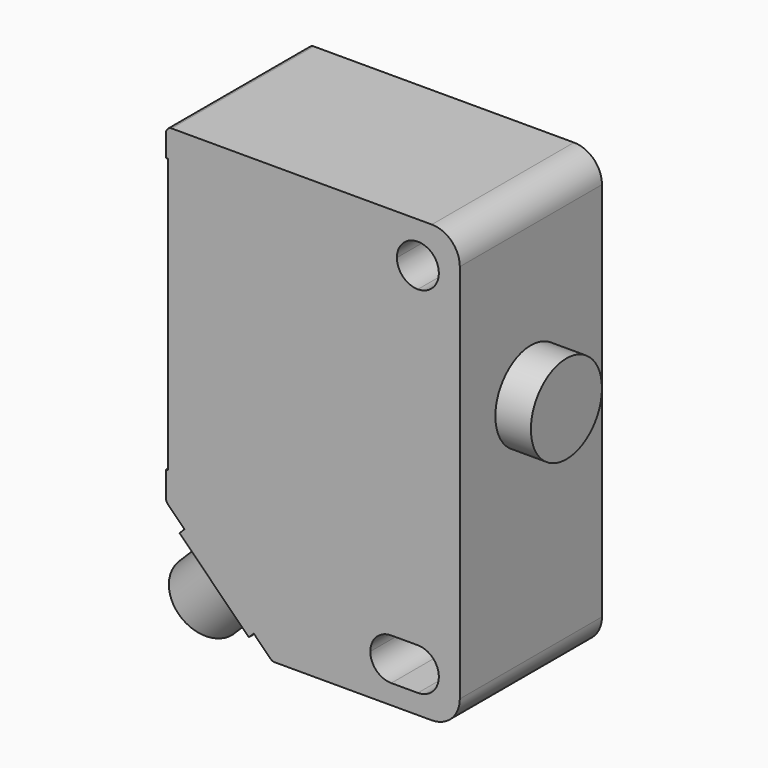
from build123d import *

# Parameters (mm, degrees)
F1_DEPTH = 12.7
F2_R     = 2.54
F3_DEPTH = 7.62
F4_R     = 3.175
F5_DEPTH = 2.54


# Not quite as in the source:
# - ends of sketch curves that miss each other by under 0.0002 mm in the source are joined


with BuildPart() as f1:
    # F0 (on Front) → F1 (new body)
    with BuildSketch(Plane.XZ):
        with BuildLine():
            Line((-46.1111856, 159.2312536), (-64.7111856, 159.2312536))
            ThreePointArc((-64.7111856, 159.2312536), (-64.9940283125, 159.1140963125), (-65.1111856, 158.8312536))
            Line((-65.1111856, 158.8312536), (-65.1111856, 157.2332636))
            Line((-65.1111856, 157.2332636), (-64.9611856, 157.2332636))
            Line((-64.9611856, 157.2332636), (-64.9611856, 137.6312536))
            Line((-64.9611856, 137.6312536), (-65.1111856, 137.6312536))
            Line((-65.1111856, 137.6312536), (-65.1111856, 135.7900576))
            ThreePointArc((-65.1111856, 135.7900576), (-65.080737413, 135.6369842271), (-64.9940283125, 135.5072148875))
            Line((-64.9940283125, 135.5072148875), (-63.7917726, 134.3049586))
            Line((-63.7917726, 134.3049586), (-64.1453256, 133.9514056))
            Line((-64.1453256, 133.9514056), (-63.6715641479, 133.4776440521))
            Line((-63.6715641479, 133.4776440521), (-59.6693400521, 129.4754191479))
            Line((-59.6693400521, 129.4754191479), (-59.1955786, 129.0016576))
            Line((-59.1955786, 129.0016576), (-58.8420246, 129.3552116))
            Line((-58.8420246, 129.3552116), (-57.6352246, 128.1484116))
            ThreePointArc((-57.6352246, 128.1484116), (-57.5054559729, 128.061701787), (-57.3523826, 128.0312536))
            Line((-57.3523826, 128.0312536), (-46.1111856, 128.0312536))
            ThreePointArc((-46.1111856, 128.0312536), (-44.6969720376, 128.6170400376), (-44.1111856, 130.0312536))
            Line((-44.1111856, 130.0312536), (-44.1111856, 134.1120546))
            Line((-44.1111856, 134.1120546), (-44.1111856, 153.1264526))
            Line((-44.1111856, 153.1264526), (-44.1111856, 156.3312536))
            Line((-44.1111856, 156.3312536), (-44.1111856, 157.2312536))
            ThreePointArc((-44.1111856, 157.2312536), (-44.6969720376, 158.6454671624), (-46.1111856, 159.2312536))
        make_face()
        with BuildLine():
            Line((-49.0111856, 132.4312536), (-47.1111856, 132.4312536))
            ThreePointArc((-47.1111856, 132.4312536), (-46.0505254282, 131.9919137718), (-45.6111856, 130.9312536))
            ThreePointArc((-45.6111856, 130.9312536), (-46.0505254282, 129.8705934282), (-47.1111856, 129.4312536))
            Line((-47.1111856, 129.4312536), (-49.0111856, 129.4312536))
            ThreePointArc((-49.0111856, 129.4312536), (-50.0718457718, 129.8705934282), (-50.5111856, 130.9312536))
            ThreePointArc((-50.5111856, 130.9312536), (-50.0718457718, 131.9919137718), (-49.0111856, 132.4312536))
        make_face(mode=Mode.SUBTRACT)
        with BuildLine():
            ThreePointArc((-47.1111856, 157.8312536), (-46.0505254282, 157.3919137718), (-45.6111856, 156.3312536))
            ThreePointArc((-45.6111856, 156.3312536), (-46.0505254282, 155.2705934282), (-47.1111856, 154.8312536))
            ThreePointArc((-47.1111856, 154.8312536), (-48.1718457718, 155.2705934282), (-48.6111856, 156.3312536))
            ThreePointArc((-48.6111856, 156.3312536), (-48.1718457718, 157.3919137718), (-47.1111856, 157.8312536))
        make_face(mode=Mode.SUBTRACT)
    extrude(amount=F1_DEPTH)

    # F2 (on face) → F3 (join)
    with BuildSketch(Plane(origin=(34.9030335203, 0, 34.9030264689), x_dir=(0, -1, 0), z_dir=(-0.7071068526, 0, -0.7071067098))):
        with Locations((6.35, 136.8855469037)):
            Circle(F2_R)
    extrude(amount=F3_DEPTH)

    # F4 (on face) → F5 (join)
    with BuildSketch(Plane.YZ.offset(-44.1111856)):
        with Locations((-6.35, 146.5312536)):
            Circle(F4_R)
    extrude(amount=F5_DEPTH)


solid = f1.part
